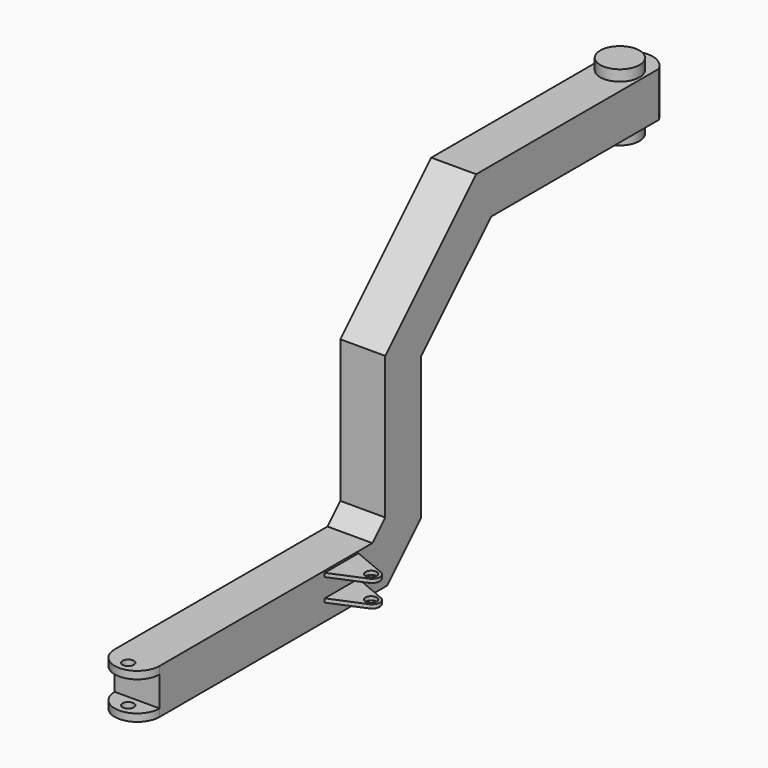
from build123d import *

# Parameters (mm, degrees)
F1_DEPTH  = 120
F2_R      = 15
F3_DEPTH  = 20
F6_DEPTH  = 120
F7_DEPTH  = 29
F8_DEPTH  = 150
F11_R     = 15
F12_DEPTH = 10


# Not quite as in the source:
# - a pattern or mirror of a feature is missing from the dataset's text; its kind, count and spacing are read off the source's solid


with BuildPart() as f1:
    # F0 (on Right) → F1 (new body)
    with BuildSketch(Plane.YZ):
        Polygon((0, 120), (0, 0), (700, 0), (760, 0), (873.1370849898, 113.1370849898), (873.1370849898, 493.1370849898), (1106.4823227814, 726.4823227814), (1556.4823227814, 726.4823227814), (1556.4823227814, 846.4823227814), (1056.7766952966, 846.4823227814), (753.1370849898, 542.8427124746), (753.1370849898, 162.8427124746), (710.2943725152, 120), (700, 120), align=None)
    extrude(amount=-F1_DEPTH)

    # F2 (on face) → F3 (join)
    with BuildSketch(Plane.XY.offset(120)):
        with BuildLine():
            Line((0, 0), (-120, 0))
            ThreePointArc((-120, 0), (-60, -60), (0, 0))
        make_face()
        with Locations((-60, -30)):
            Circle(F2_R, mode=Mode.SUBTRACT)
    f3 = extrude(amount=-F3_DEPTH)

    # F3_copies: F3 across plane
    add(f3.mirror(Plane(origin=(0, 0, 60), x_dir=(-1, 0, 0), z_dir=(0, 0, -1))))

    # F5 (on face) → F6 (join)
    with BuildSketch(Plane.XY.offset(846.4823227814)):
        Polygon((-120, 1556.4823227814), (-60, 1556.4823227814), (0, 1556.4823227814), (0, 1666.4823227814), (-120, 1666.4823227814), align=None)
        with BuildLine():
            ThreePointArc((-7.5, 1611.4823227814), (-22.8768939877, 1574.3592167691), (-60, 1558.9823227814))
            ThreePointArc((-60, 1558.9823227814), (-97.1231060123, 1648.6054287937), (-7.5, 1611.4823227814))
        make_face(mode=Mode.SUBTRACT)
        with BuildLine():
            ThreePointArc((-7.5, 1611.4823227814), (-97.1231060123, 1648.6054287937), (-60, 1558.9823227814))
            ThreePointArc((-60, 1558.9823227814), (-22.8768939877, 1574.3592167691), (-7.5, 1611.4823227814))
        make_face()
        with BuildLine():
            Line((-120, 1666.4823227814), (0, 1666.4823227814))
            ThreePointArc((0, 1666.4823227814), (-60, 1703.8881069987), (-120, 1666.4823227814))
        make_face()
    extrude(amount=-F6_DEPTH)

    # F5 (on face) → F7 (join)
    with BuildSketch(Plane.XY.offset(846.4823227814)):
        with BuildLine():
            ThreePointArc((-7.5, 1611.4823227814), (-97.1231060123, 1648.6054287937), (-60, 1558.9823227814))
            ThreePointArc((-60, 1558.9823227814), (-22.8768939877, 1574.3592167691), (-7.5, 1611.4823227814))
        make_face()
    extrude(amount=F7_DEPTH)

    # F5 (on face) → F8 (join)
    with BuildSketch(Plane.XY.offset(846.4823227814)):
        with BuildLine():
            ThreePointArc((-7.5, 1611.4823227814), (-97.1231060123, 1648.6054287937), (-60, 1558.9823227814))
            ThreePointArc((-60, 1558.9823227814), (-22.8768939877, 1574.3592167691), (-7.5, 1611.4823227814))
        make_face()
    extrude(amount=-F8_DEPTH)

    # F11 (on offset) → F12 (join)
    with BuildSketch(Plane.XY.offset(115)):
        with BuildLine():
            Line((89.2130512357, 626.3729619547), (-2.970210975, 665.1317824757))
            Line((-2.970210975, 665.1317824757), (-2.970210975, 549.5901644294))
            Line((-2.970210975, 549.5901644294), (89.2130512357, 588.3489849504))
            ThreePointArc((89.2130512357, 588.3489849504), (101.8435068324, 607.3609734525), (89.2130512357, 626.3729619547))
        make_face()
        with Locations((79.0183379768, 607.3609734525)):
            Circle(F11_R, mode=Mode.SUBTRACT)
    f12 = extrude(amount=-F12_DEPTH)

    # F12_copies: F12 across plane
    add(f12.mirror(Plane(origin=(0, 0, 80), x_dir=(-1, 0, 0), z_dir=(0, 0, -1))))


solid = f1.part
